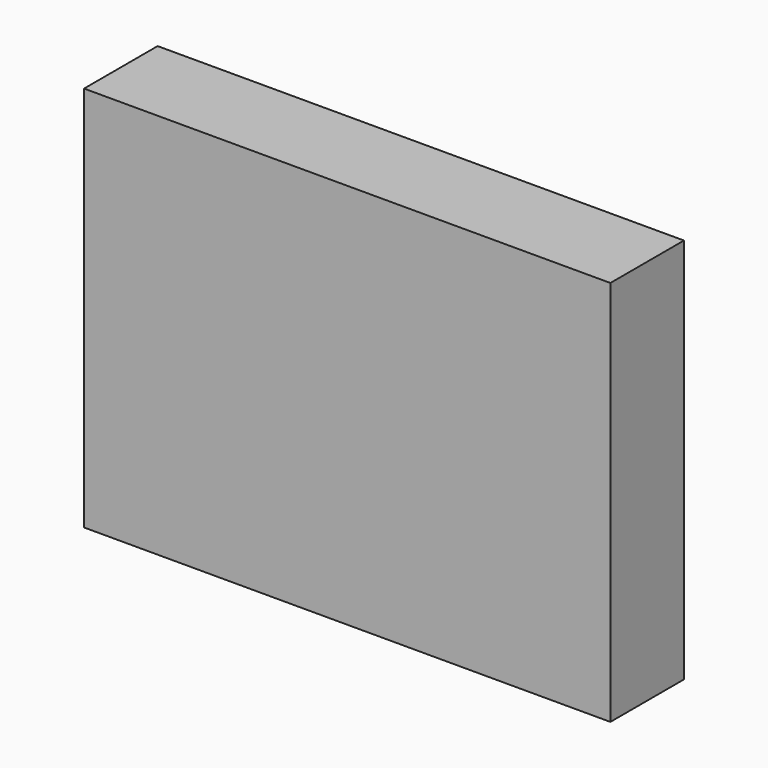
from build123d import *

# Parameters (mm, degrees)
F0_W     = 145.3452408314
F0_H     = 106.7099869251
F1_DEPTH = 25.4


# Not quite as in the source:
# - the program builds the solid bodies; features that only make, move or delete a surface that nothing else refers to are left out


with BuildPart() as f1:
    # F0 (on Front) → F1 (new body)
    with BuildSketch(Plane.XZ):
        Rectangle(F0_W, F0_H)
    extrude(amount=F1_DEPTH)


solid = f1.part
